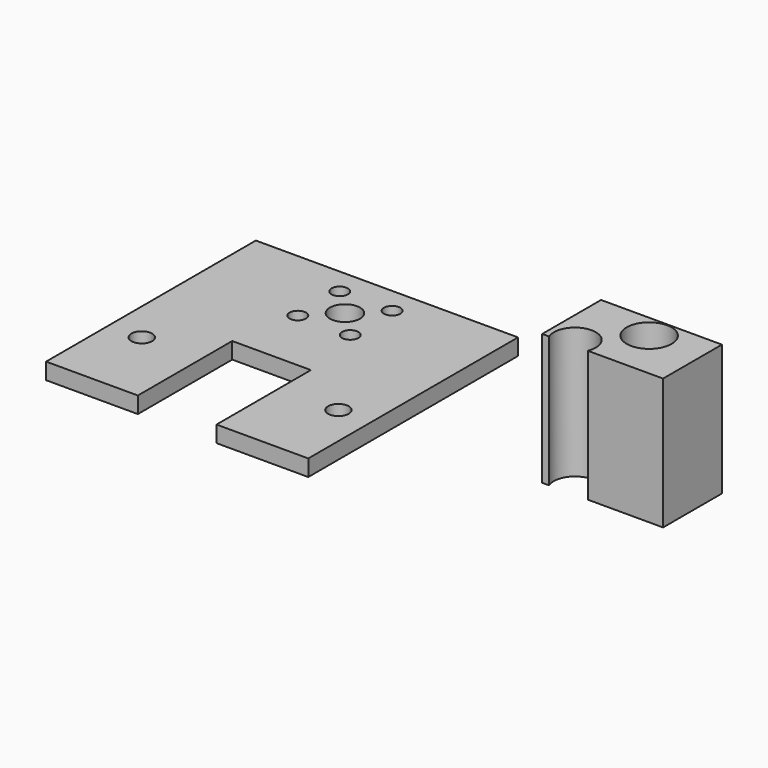
from build123d import *

# Parameters (mm, degrees)
F0_R     = 2
F0_R_2   = 1.5875
F0_R_3   = 2.921
F1_DEPTH = 3.175
F0_R_4   = 4.3534644144
F2_DEPTH = 25.4


# Not quite as in the source:
# - a feature names something its author has since deleted; it is built from what else it names


with BuildPart() as f1:
    # F0 (on Top) → F1 (new body)
    with BuildSketch(Plane.XY):
        Polygon((-25.4, 76.2436284547), (-25.4, 25.4436284547), (-7.62, 25.4436284547), (-7.62, 48.3036284547), (7.62, 48.3036284547), (7.62, 25.4436284547), (25.4, 25.4436284547), (25.4, 76.2436284547), align=None)
        with Locations((-19.05, 40.6836284547)):
            Circle(F0_R, mode=Mode.SUBTRACT)
        with Locations((19.05, 40.6836284547)):
            Circle(F0_R, mode=Mode.SUBTRACT)
        with Locations((-5.08, 61.0036284547)):
            Circle(F0_R_2, mode=Mode.SUBTRACT)
        with Locations((5.08, 61.0036284547)):
            Circle(F0_R_2, mode=Mode.SUBTRACT)
        with Locations((0, 66.0836284547)):
            Circle(F0_R_3, mode=Mode.SUBTRACT)
        with Locations((-5.08, 71.1636284547)):
            Circle(F0_R_2, mode=Mode.SUBTRACT)
        with Locations((5.08, 71.1636284547)):
            Circle(F0_R_2, mode=Mode.SUBTRACT)
    extrude(amount=F1_DEPTH)


with BuildPart() as f2:
    # F0 (on Top) → F2 (new body)
    with BuildSketch(Plane.XY):
        with BuildLine():
            Line((77.6375979185, 60.3312589228), (54.219044745, 60.3312589228))
            Line((54.219044745, 60.3312589228), (54.219044745, 46.0764877498))
            Line((54.219044745, 46.0764877498), (55.5586186913, 46.0764877498))
            ThreePointArc((55.5586186913, 46.0764877498), (58.5174025864, 51.6139923023), (63.370874914, 47.6312589228))
            ThreePointArc((63.370874914, 47.6312589228), (63.2927672969, 46.8386275918), (63.0614491436, 46.0764877498))
            Line((63.0614491436, 46.0764877498), (77.6375979185, 46.0764877498))
            Line((77.6375979185, 46.0764877498), (77.6375979185, 60.3312589228))
        make_face()
        with Locations((67.2010704875, 55.7493679225)):
            Circle(F0_R_4, mode=Mode.SUBTRACT)
    extrude(amount=F2_DEPTH)


solid = Compound([f1.part, f2.part])
